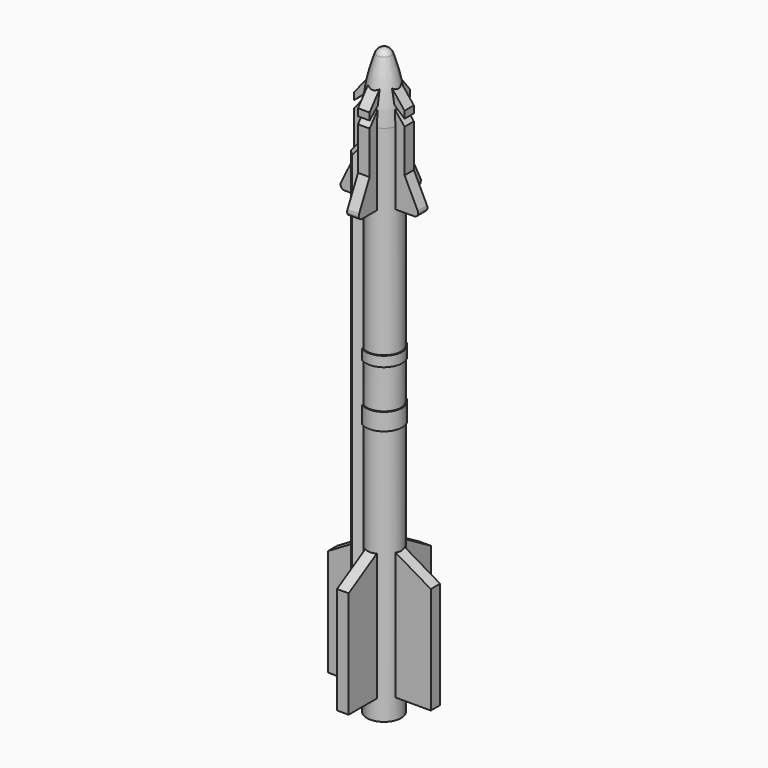
from build123d import *

# Parameters (mm, degrees)
F1_W         = 0.0347222222
F1_H         = 0.5902777778
F1_H_2       = 0.3472222222
F4_DEPTH     = 0.2
F5_COUNT     = 4
F8_DEPTH     = 16.7708333333
F9_T4_DEPTH  = 1.0631715631
F9_S5_R      = 0.5902777778
F9_T6_DEPTH  = 2
F9_T11_DEPTH = 1.0631715631
F9_S12_R     = 0.5902777778
F9_T13_DEPTH = 2


# Not quite as in the source:
# - a fillet or chamfer that OpenCascade refuses, or shapes differently, is made with other operations: its cross-section is extruded or revolved along the edge and cut away or added
# - a feature names something its author has since deleted; it is built from what else it names


with BuildPart() as f2:
    # F1 (on Front) → F2 (revolve)
    with BuildSketch(Plane.XZ):
        with Locations((0.6076388889, 9.1145833333)):
            Rectangle(F1_W, F1_H)
        with BuildLine():
            Line((0, 20.1388888889), (0, 0))
            Line((0, 0), (0.5902777778, 0))
            Line((0.5902777778, 0), (0.5902777778, 8.8194444444))
            Line((0.5902777778, 8.8194444444), (0.5902777778, 9.4097222222))
            Line((0.5902777778, 9.4097222222), (0.5902777778, 10.7638888889))
            Line((0.5902777778, 10.7638888889), (0.5902777778, 11.1111111111))
            Line((0.5902777778, 11.1111111111), (0.5902777778, 17.9861111111))
            ThreePointArc((0.5902777778, 17.9861111111), (0.5037152583, 18.9905050166), (0.2465805636, 19.9652777778))
            ThreePointArc((0.2465805636, 19.9652777778), (0.1507836134, 20.0911322234), (0, 20.1388888889))
        make_face()
        with Locations((0.6076388889, 10.9375)):
            Rectangle(F1_W, F1_H_2)
    revolve(axis=Axis((0, 0, 10.0694444444), (0, 0, 1)))

    # F3 (on Front) → F4 (join, symmetric)
    with BuildSketch(Plane.XZ):
        with BuildLine():
            Line((0, 19.6614583333), (0, 0.6944444444))
            Line((0, 0.6944444444), (1.7708333333, 0.6944444444))
            Line((1.7708333333, 0.6944444444), (1.7708333333, 4.375))
            Line((1.7708333333, 4.375), (0.4, 5.181372549))
            Line((0.4, 5.181372549), (0.4, 15.4861111111))
            Line((0.4, 15.4861111111), (1.1979166667, 15.4861111111))
            ThreePointArc((1.1979166667, 15.4861111111), (1.3157028026, 15.5514027878), (1.3227463965, 15.685890574))
            Line((1.3227463965, 15.685890574), (0.8680555556, 16.618037065))
            Line((0.8680555556, 16.618037065), (0.2, 17.9875954237))
            Line((0.2, 17.9875954237), (0.2, 18.0570398682))
            Line((0.2, 18.0570398682), (0.8680555556, 16.6874815094))
            Line((0.8680555556, 16.6874815094), (0.8680555556, 18.0902777778))
            Line((0.8680555556, 18.0902777778), (0.2199074074, 18.900462963))
            Line((0.2199074074, 18.900462963), (0.8680555556, 18.3333333333))
            Line((0.8680555556, 18.3333333333), (0.8680555556, 18.5763888889))
            Line((0.8680555556, 18.5763888889), (0, 19.6614583333))
        make_face()
        Polygon((0.2, 18.9253472222), (0.2199074074, 18.900462963), (0.2, 18.9178819444), align=None, mode=Mode.SUBTRACT)
        Polygon((0.8680555556, 16.618037065), (0.8680555556, 16.6874815094), (0.2, 18.0570398682), (0.2, 17.9875954237), align=None)
        Polygon((0.2, 18.9178819444), (0.2199074074, 18.900462963), (0.2, 18.9253472222), align=None)
    extrude(amount=F4_DEPTH, both=True)

    # F5: F2 ×4 about axis
    f5_axis = Axis((0, 0, 8.8194444444), (0, 0, 1))


with BuildPart() as f2_1:
    add(f2.part)
    for i in range(1, F5_COUNT):
        add(f2.part.rotate(f5_axis, i * 360 / F5_COUNT))

    # F7 (on offset) → F8 (join)
    with BuildSketch(Plane.XY.offset(0.5208333333)):
        Polygon((-0.5205091584, -0.7267486362), (-0.0531495446, -0.2593890224), (-0.2593890224, -0.0531495446), (-0.7267486362, -0.5205091584), align=None)
    extrude(amount=F8_DEPTH)

    # F9: chamfer of 0.3 on 2 edges, made by hand


with BuildPart() as f9_tool2:
    # F9_s3 → F9_t4 (new body)
    with BuildSketch(Plane(origin=(-0.1031197389, 0.1031197389, 0), x_dir=(0, 0, 1), z_dir=(0.7071067812, -0.7071067812, 0))):
        Polygon((0.8208333333, 0.8819444444), (0.5208333333, 0.5819444444), (0.5208333333, 0.8819444444), align=None)
    extrude(amount=F9_T4_DEPTH)

    # F9_s5 → F9_t6 (cut, symmetric)
    with BuildSketch(Plane.XY.offset(0.7)):
        Circle(F9_S5_R)
    extrude(amount=F9_T6_DEPTH, both=True, mode=Mode.SUBTRACT)

    split(bisect_by=Plane.YZ.offset(-0.2), keep=Keep.BOTTOM)


with BuildPart() as f2_2:
    add(f2_1.part)

    # F9_t1: cut F9_tool2
    add(f9_tool2.part, mode=Mode.SUBTRACT)


with BuildPart() as f9_tool9:
    # F9_s10 → F9_t11 (new body)
    with BuildSketch(Plane(origin=(-0.1031197389, 0.1031197389, 0), x_dir=(0, 0, 1), z_dir=(0.7071067812, -0.7071067812, 0))):
        Polygon((16.9916666667, 0.8819444444), (17.2916666667, 0.5819444444), (17.2916666667, 0.8819444444), align=None)
    extrude(amount=F9_T11_DEPTH)

    # F9_s12 → F9_t13 (cut, symmetric)
    with BuildSketch(Plane.XY.offset(17.1)):
        Circle(F9_S12_R)
    extrude(amount=F9_T13_DEPTH, both=True, mode=Mode.SUBTRACT)

    split(bisect_by=Plane.YZ.offset(-0.2), keep=Keep.BOTTOM)


with BuildPart() as f2_3:
    add(f2_2.part)

    # F9_t8: cut F9_tool9
    add(f9_tool9.part, mode=Mode.SUBTRACT)


solid = f2_3.part
